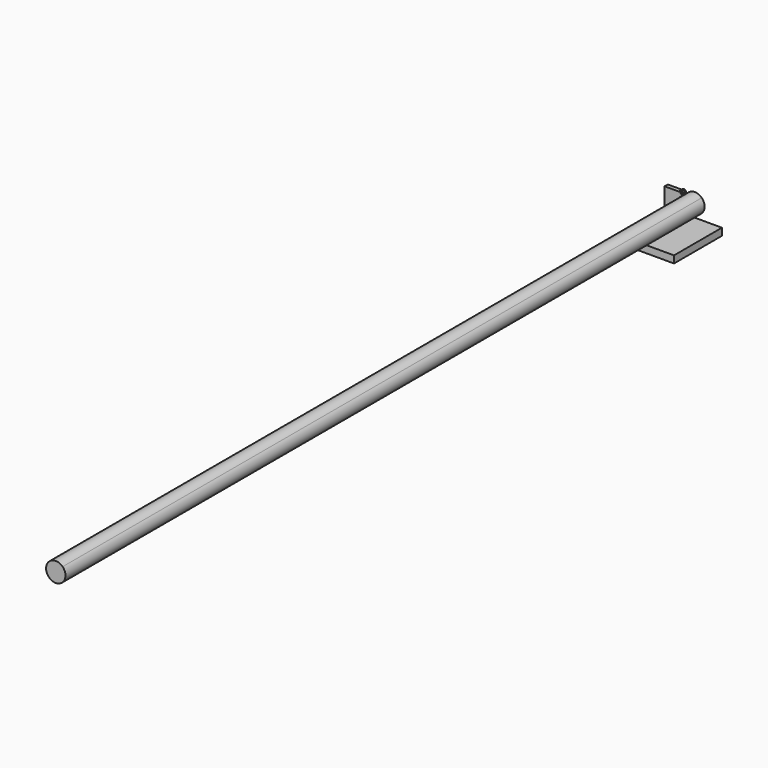
from build123d import *

# Parameters (mm, degrees)
F1_DEPTH  = 2000
F2_DEPTH  = 10
F3_R      = 2.5
F4_DEPTH  = 25
F5_R      = 2.5
F6_DEPTH  = 25
F7_DEPTH  = 150
F9_DEPTH  = 10
F10_DEPTH = 25
F11_R     = 4.99999


# Not quite as in the source:
# - a fillet or chamfer is up to 0.001 mm smaller than in the source, because OpenCascade refuses the exact size


with BuildPart() as f1:
    # F0 (on Front) → F1 (new body)
    with BuildSketch(Plane.XZ):
        with BuildLine():
            ThreePointArc((17.1826947828, -17.1826947828), (22.45027264, -9.2992074065), (24.3, 0))
            ThreePointArc((24.3, 0), (22.45027264, 9.2992074065), (17.1826947828, 17.1826947828))
            ThreePointArc((17.1826947828, 17.1826947828), (0, 24.3), (-17.1826947828, 17.1826947828))
            ThreePointArc((-17.1826947828, 17.1826947828), (-24.3, 0), (-17.1826947828, -17.1826947828))
            ThreePointArc((-17.1826947828, -17.1826947828), (0, -24.3), (17.1826947828, -17.1826947828))
        make_face()
    extrude(amount=F1_DEPTH)


with BuildPart() as f2:
    # F0 (on Front) → F2 (new body)
    with BuildSketch(Plane.XZ):
        Polygon((-35, 2.1938166904), (-23.9002092041, 13.2936074863), (-30.971277016, 20.3646752982), (-32.360868023, 18.9750842911), (-35, 16.3359523141), align=None)
        Polygon((-35, 16.3359523141), (-32.360868023, 18.9750842911), (-35, 18.9750842911), align=None)
        Polygon((-35, -2.1938166904), (-35, 2.1938166904), (-35, 16.3359523141), (-35, 18.9750842911), (-67.6910728216, 18.9750842911), (-67.6910728216, -32.3), (-35, -32.3), (-35, -20.3646752982), (-35, -16.3359523141), align=None)
        Polygon((-23.9002092041, -13.2936074863), (-35, -2.1938166904), (-35, -16.3359523141), (-30.971277016, -20.3646752982), align=None)
        Polygon((-30.971277016, -20.3646752982), (-35, -16.3359523141), (-35, -20.3646752982), align=None)
    extrude(amount=F2_DEPTH)

    # F3 (on face) → F4 (cut)
    with BuildSketch(Plane(origin=(-5.3033008589, 0, -5.3033008589), x_dir=(0, 1, 0), z_dir=(0.7071067812, 0, 0.7071067812))):
        with Locations((-5, 31.3)):
            Circle(F3_R)
    extrude(amount=-F4_DEPTH, mode=Mode.SUBTRACT)

    # F5 (on face) → F6 (cut)
    with BuildSketch(Plane(origin=(-5.3033008589, 0, 5.3033008589), x_dir=(0, 1, 0), z_dir=(0.7071067812, 0, -0.7071067812))):
        with Locations((-5, -31.3)):
            Circle(F5_R)
    extrude(amount=-F6_DEPTH, mode=Mode.SUBTRACT)


with BuildPart() as f7:
    # F0 (on Front) → F7 (new body)
    with BuildSketch(Plane.XZ):
        Polygon((-35, -32.3), (-67.6910728216, -32.3), (-67.6910728216, -50.238545984), (0, -50.238545984), (0, -32.3), align=None)
    extrude(amount=F7_DEPTH)

    # F8: F7 across face


with BuildPart() as f7_1:
    add(f7.part)
    add(f7.part.mirror(Plane(origin=(0, -75, -41.269272992), x_dir=(0, 1, 0), z_dir=(1, 0, 0))))


with BuildPart() as f9:
    # F0 (on Front) → F9 (new body)
    with BuildSketch(Plane.XZ):
        Polygon((-23.9002092041, 13.2936074863), (-20.3646752982, 16.8291413922), (-27.43574311, 23.9002092041), (-30.971277016, 20.3646752982), align=None)
    extrude(amount=F9_DEPTH)

    # F3 (on face) → F10 (cut)
    with BuildSketch(Plane(origin=(-5.3033008589, 0, -5.3033008589), x_dir=(0, 1, 0), z_dir=(0.7071067812, 0, 0.7071067812))):
        with Locations((-5, 31.3)):
            Circle(F3_R)
    extrude(amount=F10_DEPTH, mode=Mode.SUBTRACT)

    # F11 (radius 5 in the source; OpenCascade refuses exactly that, so slightly less here)
    f11_edges = [f9.edges().sort_by_distance(p)[0] for p in [
        (-29.20351, 0, 22.132442),
        (-29.20351, -10, 22.132442),
        (-22.132442, -10, 15.061374),
        (-22.132442, 0, 15.061374),
    ]]
    fillet(f11_edges, radius=F11_R)


solid = Compound([f1.part, f2.part, f7_1.part, f9.part])
